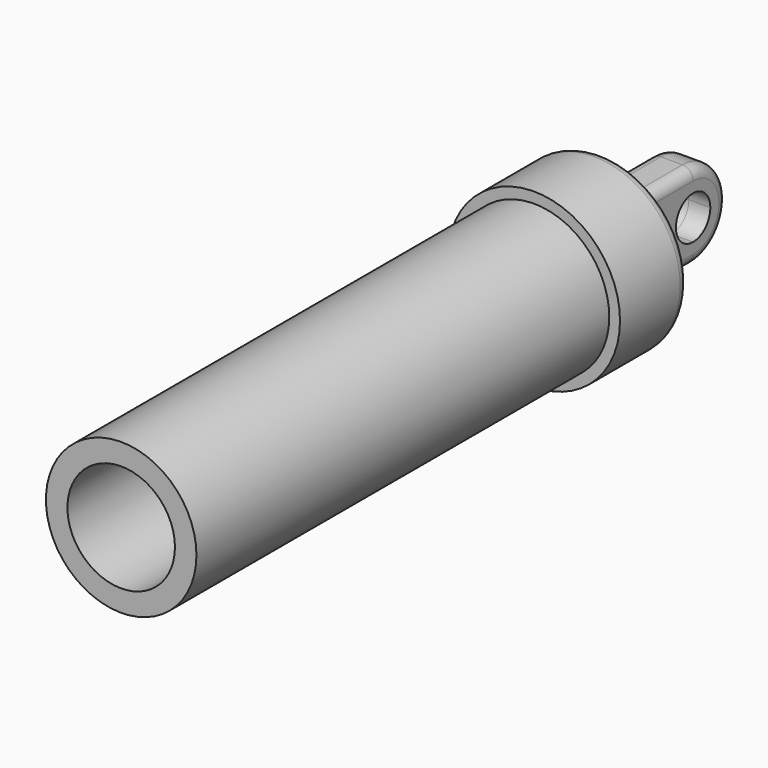
from build123d import *

# Parameters (mm, degrees)
F0_R     = 12.7
F1_DEPTH = 12.7
F3_DEPTH = 3.175
F4_F1_R  = 1.5875
F4_F2_R  = 1.5875
F5_R     = 11.1125
F6_DEPTH = 76.2
F7_R     = 7.9375
F8_DEPTH = 76.2


with BuildPart() as f1:
    # F0 (on Front) → F1 (new body)
    with BuildSketch(Plane.XZ):
        Circle(F0_R)
    extrude(amount=F1_DEPTH)

    # F2 (on Right) → F3 (join, symmetric)
    with BuildSketch(Plane.YZ):
        with BuildLine():
            Line((0, 6.35), (0, -6.35))
            Line((0, -6.35), (12.7, -6.35))
            ThreePointArc((12.7, -6.35), (6.35, 0), (12.7, 6.35))
            Line((12.7, 6.35), (0, 6.35))
        make_face()
        with BuildLine():
            ThreePointArc((12.7, 6.35), (6.35, 0), (12.7, -6.35))
            Line((12.7, -6.35), (12.7, -3.175))
            ThreePointArc((12.7, -3.175), (9.525, 0), (12.7, 3.175))
            Line((12.7, 3.175), (12.7, 6.35))
        make_face()
        with BuildLine():
            Line((12.7, -3.175), (12.7, -6.35))
            ThreePointArc((12.7, -6.35), (17.1901280605, -4.4901280605), (19.05, 0))
            ThreePointArc((19.05, 0), (17.1901280605, 4.4901280605), (12.7, 6.35))
            Line((12.7, 6.35), (12.7, 3.175))
            ThreePointArc((12.7, 3.175), (14.9450640303, 2.2450640303), (15.875, 0))
            ThreePointArc((15.875, 0), (14.9450640303, -2.2450640303), (12.7, -3.175))
        make_face()
    extrude(amount=F3_DEPTH, both=True)

    # F4: fillet of radius 1.5875 on 10 edges, made by hand

    # F4_f1
    f4_f1_edges = [f1.edges().sort_by_distance(p)[0] for p in [
        (-12.7, 0, 0),
        (3.175, 6.35, 6.35),
        (-3.175, 6.35, 6.35),
        (-3.175, 6.35, -6.35),
        (-3.175, 19.05, 0),
        (3.175, 6.35, -6.35),
        (3.175, 19.05, 0),
    ]]
    fillet(f4_f1_edges, radius=F4_F1_R)

    # F4_f2
    f4_f2_edges = [f1.edges().sort_by_distance(p)[0] for p in [
        (-3.175, 0, 0),
        (0, 0, 6.35),
        (3.175, 0, 0),
        (2.7100320151, 0, 5.8850320151),
        (2.7100320151, 0, -5.8850320151),
        (-2.7100320151, 0, 5.8850320151),
        (-2.7100320151, 0, -5.8850320151),
    ]]
    fillet(f4_f2_edges, radius=F4_F2_R)


with BuildPart() as f6:
    # F5 (on face) → F6 (new body)
    with BuildSketch(Plane.XZ.offset(12.7)):
        Circle(F5_R)
    extrude(amount=F6_DEPTH)

    # F7 (on face) → F8 (cut)
    with BuildSketch(Plane.XZ.offset(88.9)):
        Circle(F7_R)
    extrude(amount=-F8_DEPTH, mode=Mode.SUBTRACT)


solid = Compound([f1.part, f6.part])
